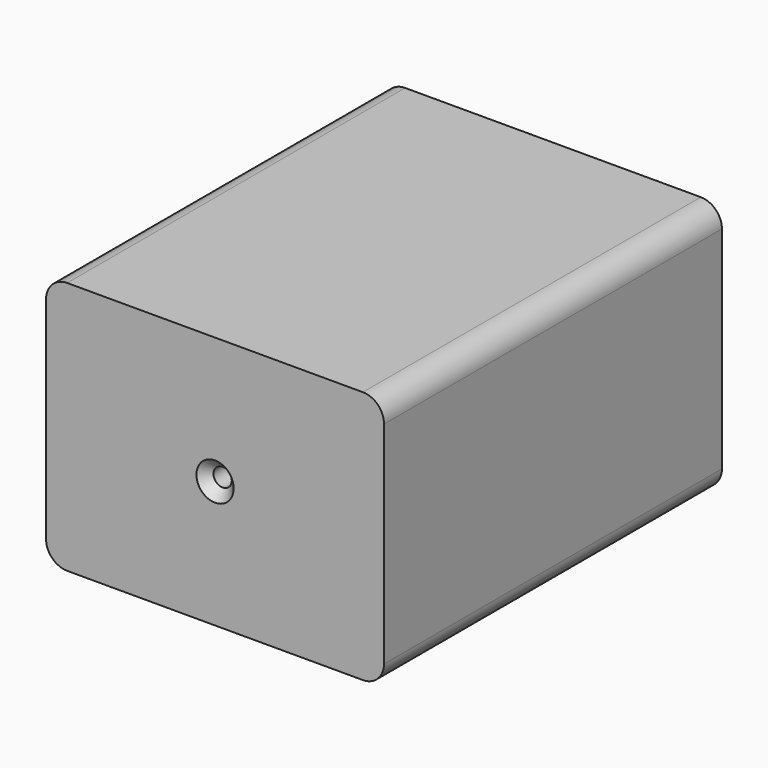
from build123d import *

# Parameters (mm, degrees)
F1_DEPTH       = 127
F3_D           = 5.5
F3_DEPTH       = 12.7
F3_CSINK_D     = 11.2
F3_CSINK_ANGLE = 90
F3_TIP         = 1.6523667023


with BuildPart() as f1:
    # F0 (on Front) → F1 (new body)
    with BuildSketch(Plane.XZ):
        with BuildLine():
            ThreePointArc((-50.8, -31.75), (-48.9401280605, -36.2401280605), (-44.45, -38.1))
            Line((-44.45, -38.1), (44.45, -38.1))
            ThreePointArc((44.45, -38.1), (48.9401280605, -36.2401280605), (50.8, -31.75))
            Line((50.8, -31.75), (50.8, 31.75))
            ThreePointArc((50.8, 31.75), (48.9401280605, 36.2401280605), (44.45, 38.1))
            Line((44.45, 38.1), (-44.45, 38.1))
            ThreePointArc((-44.45, 38.1), (-48.9401280605, 36.2401280605), (-50.8, 31.75))
            Line((-50.8, 31.75), (-50.8, -31.75))
        make_face()
    extrude(amount=F1_DEPTH)

    # F3
    with Locations(Plane.XZ.offset(127)):
        with Locations((0, 0)):
            CounterSinkHole(F3_D / 2, F3_CSINK_D / 2, depth=F3_DEPTH, counter_sink_angle=F3_CSINK_ANGLE)
            with Locations((0, 0, -(F3_DEPTH + F3_TIP / 2))):  # 118° drill point
                Cone(0, F3_D / 2, F3_TIP, mode=Mode.SUBTRACT)


solid = f1.part
